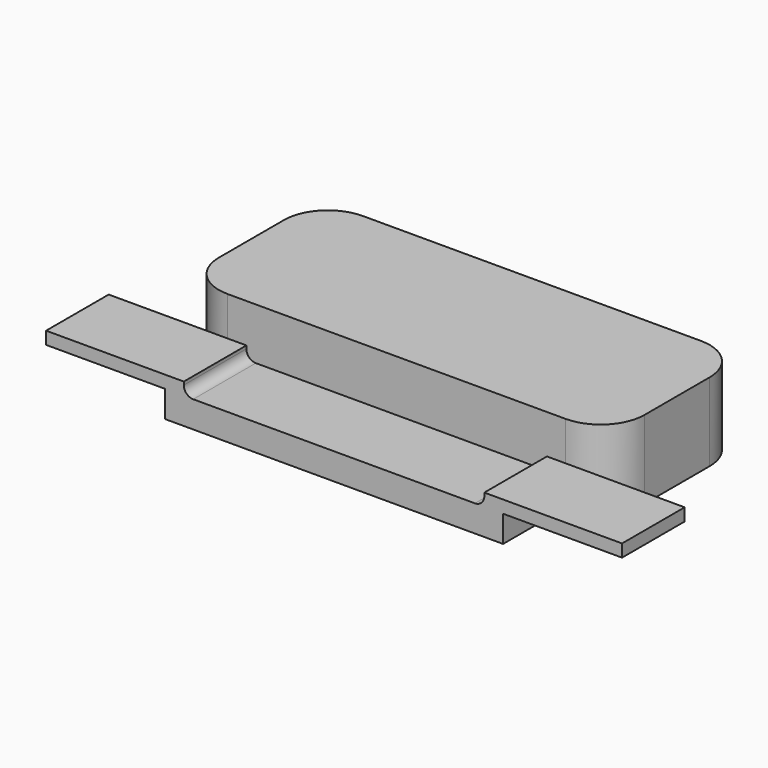
from build123d import *

# Parameters (mm, degrees)
F1_DEPTH = 12.5
F5_DEPTH = 25


# Not quite as in the source:
# - the program builds the solid bodies; features that only make, move or delete a surface that nothing else refers to are left out


with BuildPart() as f1:
    # F0 (on Top) → F1 (new body, symmetric)
    with BuildSketch(Plane.XY):
        with BuildLine():
            Line((-122, 0), (-14, 0))
            ThreePointArc((-14, 0), (-4.1005050634, 4.1005050634), (0, 14))
            Line((0, 14), (0, 40))
            ThreePointArc((0, 40), (-4.1005050634, 49.8994949366), (-14, 54))
            Line((-14, 54), (-122, 54))
            ThreePointArc((-122, 54), (-131.8994949366, 49.8994949366), (-136, 40))
            Line((-136, 40), (-136, 14))
            ThreePointArc((-136, 14), (-131.8994949366, 4.1005050634), (-122, 0))
        make_face()
    extrude(amount=F1_DEPTH, both=True)

    # F4 (on face) → F5 (join)
    with BuildSketch(Plane.XZ):
        with BuildLine():
            Line((-122, -4), (-122, -12.5))
            Line((-122, -12.5), (-14, -12.5))
            Line((-14, -12.5), (-14, -4))
            Line((-14, -4), (24, -4))
            Line((24, -4), (24, 0))
            Line((24, 0), (-20, 0))
            Line((-20, 0), (-20, -1))
            ThreePointArc((-20, -1), (-20.8786796564, -3.1213203436), (-23, -4))
            Line((-23, -4), (-113, -4))
            ThreePointArc((-113, -4), (-115.1213203436, -3.1213203436), (-116, -1))
            Line((-116, -1), (-116, 0))
            Line((-116, 0), (-160, 0))
            Line((-160, 0), (-160, -4))
            Line((-160, -4), (-122, -4))
        make_face()
    extrude(amount=F5_DEPTH)


solid = f1.part
